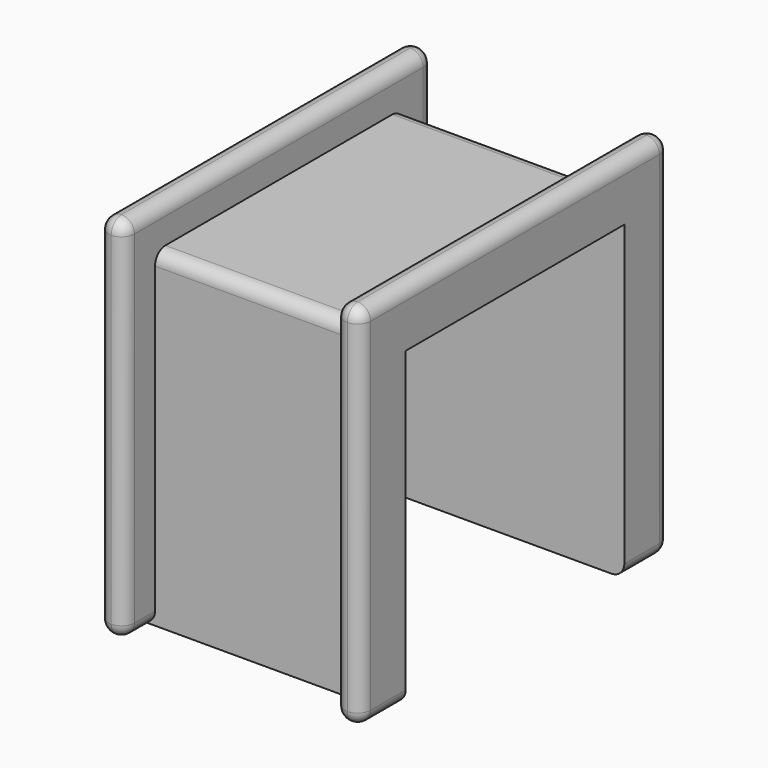
from build123d import *

# Parameters (mm, degrees)
F0_W     = 10.16
F0_H     = 15
F1_DEPTH = 14.28
F2_W     = 8.16
F2_H     = 14.28
F5_DEPTH = 1.5
F3_W     = 8.16
F3_H     = 15
F6_DEPTH = 1.5
F4_W     = 8.16
F4_H     = 14.28
F7_DEPTH = 1.5
F8_W     = 10.6
F8_H     = 12.08
F9_DEPTH = 25
F10_R    = 0.49999


# Not quite as in the source:
# - a fillet or chamfer is up to 0.001 mm smaller than in the source, because OpenCascade refuses the exact size


with BuildPart() as f1:
    # F0 (on Top) → F1 (new body)
    with BuildSketch(Plane.XY):
        Rectangle(F0_W, F0_H)
    extrude(amount=F1_DEPTH)

    # F2 (on face) → F5 (cut)
    with BuildSketch(Plane.XZ.offset(7.5)):
        with Locations((0, 7.14)):
            Rectangle(F2_W, F2_H)
    extrude(amount=-F5_DEPTH, mode=Mode.SUBTRACT)

    # F3 (on face) → F6 (cut)
    with BuildSketch(Plane.XY.offset(14.28)):
        Rectangle(F3_W, F3_H)
    extrude(amount=-F6_DEPTH, mode=Mode.SUBTRACT)

    # F4 (on face) → F7 (cut)
    with BuildSketch(Plane(origin=(0, 7.5, 0), x_dir=(-1, 0, 0), z_dir=(0, 1, 0))):
        with Locations((0, 7.14)):
            Rectangle(F4_W, F4_H)
    extrude(amount=-F7_DEPTH, mode=Mode.SUBTRACT)

    # F8 (on face) → F9 (cut)
    with BuildSketch(Plane.YZ.offset(5.08)):
        with Locations((0, 6.04)):
            Rectangle(F8_W, F8_H)
    extrude(amount=-F9_DEPTH, mode=Mode.SUBTRACT)

    # F10 (radius 0.5 in the source; OpenCascade refuses exactly that, so slightly less here)
    f10_edges = [f1.edges().sort_by_distance(p)[0] for p in [
        (-4.58, -7.5, 14.28),
        (4.58, -7.5, 14.28),
        (-4.08, -7.5, 7.14),
        (-5.08, -7.5, 7.14),
        (-5.08, 0, 14.28),
        (-5.08, 0, 12.08),
        (-5.08, -5.3, 6.04),
        (-5.08, -6.4, 0),
        (-4.58, -7.5, 0),
        (4.58, -7.5, 0),
        (4.08, -7.5, 7.14),
        (5.08, -7.5, 7.14),
        (5.08, 0, 14.28),
        (-4.08, 0, 14.28),
        (4.08, 0, 14.28),
        (5.08, 7.5, 7.14),
        (4.08, 7.5, 7.14),
        (-4.08, 7.5, 7.14),
        (-5.08, 7.5, 7.14),
        (-4.58, 7.5, 14.28),
        (4.58, 7.5, 14.28),
        (4.58, 7.5, 0),
        (-4.58, 7.5, 0),
        (-5.08, 6.4, 0),
        (-4.08, 6.75, 0),
        (4.08, 6.75, 0),
        (5.08, 6.4, 0),
        (5.08, -6.4, 0),
        (-4.08, -6.75, 0),
        (4.08, -6.75, 0),
        (0, -6, 12.78),
        (0, 6, 12.78),
    ]]
    fillet(f10_edges, radius=F10_R)


solid = f1.part
